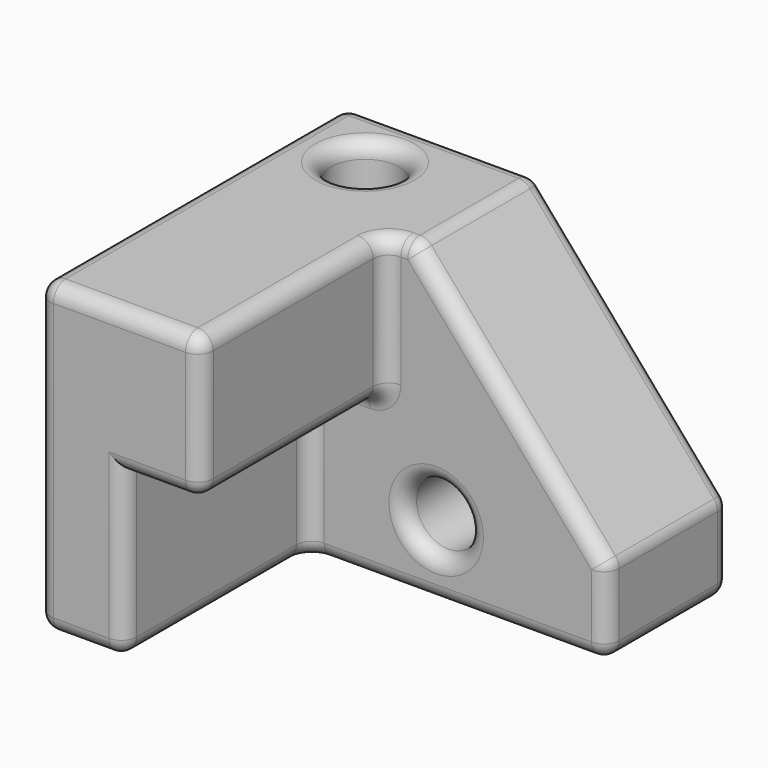
from build123d import *

# Parameters (mm, degrees)
F0_W     = 127
F0_H     = 101.6
F1_DEPTH = 127
F3_DEPTH = 76.2
F4_R     = 10.5227523194
F5_DEPTH = 50.801
F6_R     = 11.2911618422
F7_DEPTH = 101.601
F8_SIZE2 = 73.66
F8_SIZE  = 63.5
F9_R     = 5.08


with BuildPart() as f1:
    # F0 (on Front) → F1 (new body)
    with BuildSketch(Plane.XZ):
        with Locations((9.6775274724, -3.4555412512)):
            Rectangle(F0_W, F0_H)
    extrude(amount=F1_DEPTH)

    # F2 (on face) → F3 (cut)
    with BuildSketch(Plane.XZ.offset(127)):
        Polygon((73.1775274724, 47.3444587488), (0, 47.3444587488), (0, 0), (-25.3069717437, 0), (-25.3069717437, -54.2555412512), (73.1775274724, -54.2555412512), align=None)
    extrude(amount=-F3_DEPTH, mode=Mode.SUBTRACT)

    # F4 (on face) → F5 (cut, through all)
    with BuildSketch(Plane.XZ.offset(50.8)):
        with Locations((16.7653001845, -30.3956214339)):
            Circle(F4_R)
    extrude(amount=-F5_DEPTH, mode=Mode.SUBTRACT)

    # F6 (on face) → F7 (cut, through all)
    with BuildSketch(Plane.XY.offset(47.3444587488)):
        with Locations((-29.2597617954, -22.6739365608)):
            Circle(F6_R)
    extrude(amount=-F7_DEPTH, mode=Mode.SUBTRACT)

    # F8
    f8_edges = [f1.edges().sort_by_distance(p)[0] for p in [
        (73.177527, -25.4, 47.344459),
    ]]
    f8_side = f1.faces().sort_by_distance((-3.567211, -51.159815, 47.344459))[0]
    chamfer(f8_edges, length=F8_SIZE, length2=F8_SIZE2, reference=f8_side)

    # F9
    f9_edges = [f1.edges().sort_by_distance(p)[0] for p in [
        (-26.911236, -127, 47.344459),
        (-53.822473, -127, -3.455541),
        (0, -127, 23.672229),
        (-12.653486, -127, 0),
        (-25.306972, -127, -27.127771),
        (-39.564722, -127, -54.255541),
        (0, -88.9, 47.344459),
        (0, -88.9, 0),
        (0, -50.8, 23.672229),
        (-22.072473, 0, 47.344459),
        (9.677527, -25.4, 47.344459),
        (-53.822473, -63.5, 47.344459),
        (4.838764, -50.8, 47.344459),
        (-40.550924, -22.673937, 47.344459),
        (41.427527, 0, 10.514459),
        (73.177527, -25.4, -26.315541),
        (41.427527, -50.8, 10.514459),
        (73.177527, -50.8, -40.285541),
        (-12.653486, -50.8, 0),
        (23.935278, -50.8, -54.255541),
        (-25.306972, -50.8, -27.127771),
        (6.242548, -50.8, -30.395621),
        (73.177527, 0, -40.285541),
        (73.177527, -25.4, -54.255541),
        (9.677527, 0, -54.255541),
        (-53.822473, 0, -3.455541),
        (6.242548, 0, -30.395621),
        (-53.822473, -63.5, -54.255541),
        (-25.306972, -88.9, -54.255541),
    ]]
    fillet(f9_edges, radius=F9_R)


solid = f1.part
